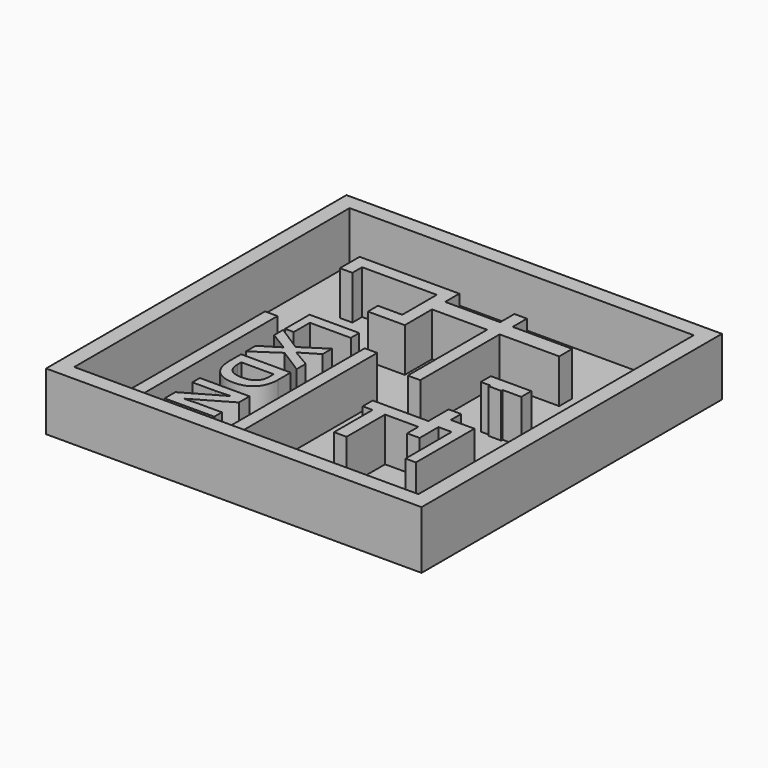
from build123d import *

# Parameters (mm, degrees)
F0_W         = 38.1
F0_H         = 38.1
F1_DEPTH     = 0.79375
F2_W         = 38.1
F2_H         = 38.1
F2_W_2       = 34.925
F2_H_2       = 34.925
F3_DEPTH     = 5.08
F4_W         = 1.27
F4_H         = 17.8449655165
F5_DEPTH     = 4.445
F6_TEXT_SIZE = 7.0555555556
F7_DEPTH     = 4.445
F4_R         = 1.27
F4_R_2       = 1.2667228734
F8_DEPTH     = 0.396875


# Not quite as in the source:
# - a feature names something its author has since deleted; it is built from what else it names
# - Text() gives the source's letters only with a copy of the font that has no kerning and outlines rounded to 1/6400 em; it was checked with that copy


with BuildPart() as f1:
    # F0 (on Top) → F1 (new body)
    with BuildSketch(Plane.XY):
        with Locations((-4.4299233705, -5.2025716019)):
            Rectangle(F0_W, F0_H)
    extrude(amount=F1_DEPTH)

    # F2 (on face) → F3 (join)
    with BuildSketch(Plane.XY.offset(0.79375)):
        with Locations((-4.4299233705, -5.2025716019)):
            Rectangle(F2_W, F2_H)
        with Locations((-4.4299233705, -5.2025716019)):
            Rectangle(F2_W_2, F2_H_2, mode=Mode.SUBTRACT)
    extrude(amount=F3_DEPTH)

    # F4 (on face) → F5 (join)
    with BuildSketch(Plane.XY.offset(0.79375)):
        with Locations((-16.1774233705, -13.7425888436)):
            Rectangle(F4_W, F4_H)
        with Locations((-6.0563569039, -13.7425888436)):
            Rectangle(F4_W, F4_H)
        Polygon((5.0506445458, -12.6968109491), (5.0506445458, -14.1183262791), (6.3206445458, -14.1183262791), (6.3206445458, -11.7316003889), (7.6602357381, -11.7316003889), (7.6602357381, -17.5850716019), (8.7145766295, -17.5850716019), (8.7145766295, -10.1658768654), (6.3206445458, -10.1658768654), (6.3206445458, -8.8519840366), (5.0506445458, -8.8519840366), (5.0506445458, -11.4268109491), (-0.5953569039, -11.4268109491), (-0.5953569039, -12.6968109491), (0.404487364, -12.6968109491), (0.404487364, -17.5850716019), (1.674487364, -17.5850716019), (1.674487364, -12.6968109491), align=None)
        Polygon((8.2065766295, -2.3156417942), (4.1016049562, -2.3156417942), (4.1016049562, -3.5856417942), (5.0506445458, -3.5856417942), (5.0506445458, -3.7719840366), (6.3206445458, -3.7719840366), (6.3206445458, -3.5856417942), (8.2065766295, -3.5856417942), align=None)
        Polygon((-15.5424233705, 4.6768859108), (-15.5424233705, 5.9099283981), (-7.9613569039, 5.9099283981), (-7.9613569039, 1.5298939146), (-10.4319751263, 1.5298939146), (-10.4319751263, 0.2598939146), (-6.6913569039, 0.2598939146), (-6.6913569039, 3.7199111564), (-1.1033569039, 3.7199111564), (-1.1033569039, -6.3468109491), (0.1666430961, -6.3468109491), (0.1666430961, 3.7199111564), (6.21287385, 3.7199111564), (6.21287385, 5.3709111564), (0.1666430961, 5.3709111564), (0.1666430961, 7.1799283981), (-1.1033569039, 7.1799283981), (-1.1033569039, 5.3709111564), (-6.6913569039, 5.3709111564), (-6.6913569039, 7.1799283981), (-16.8124233705, 7.1799283981), (-16.8124233705, 4.6768859108), align=None)
    extrude(amount=F5_DEPTH)

    # F6 (on face) → F7 (join)
    with BuildSketch(Plane.XY.offset(0.79375)):
        with Locations(Location((-13.7056577039, -2.4137230015), (0, 0, -90))):
            Text('LXDN', F6_TEXT_SIZE, font='Open Sans', font_style=FontStyle.BOLD, text_align=(TextAlign.LEFT, TextAlign.BOTTOM))
    extrude(amount=F7_DEPTH)

    # F4 (on face) → F8 (cut)
    with BuildSketch(Plane.XY.offset(0.79375)):
        with Locations((-19.3524233705, -18.903022632)):
            Circle(F4_R)
        with Locations((10.8735766295, -20.3813277185)):
            Circle(F4_R_2)
    extrude(amount=-F8_DEPTH, mode=Mode.SUBTRACT)


solid = f1.part
